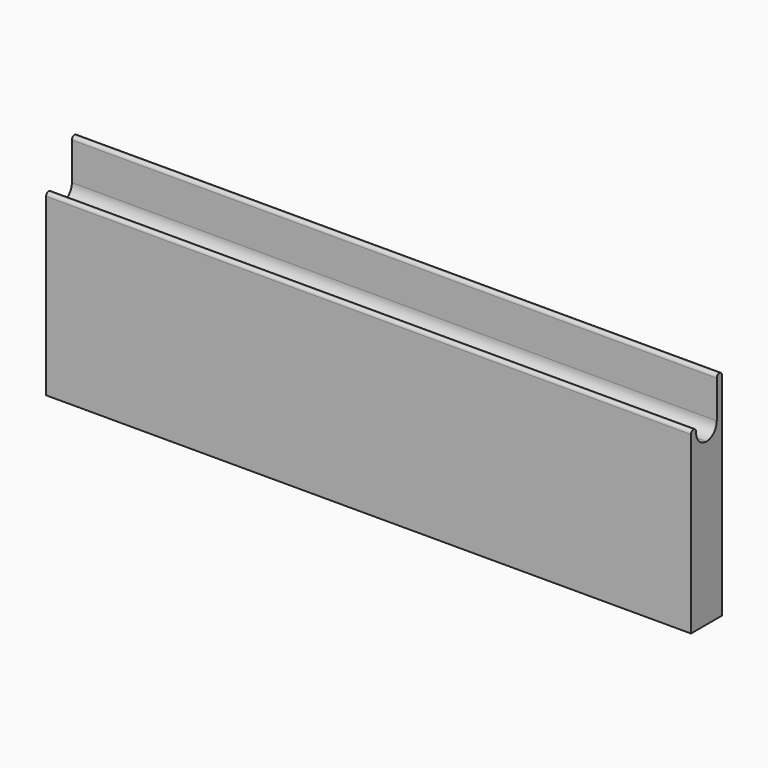
from build123d import *

# Parameters (mm, degrees)
F0_W     = 300
F0_H     = 100
F1_DEPTH = 9
F3_DEPTH = 300.001
F4_R     = 1.49999
F5_R     = 5.99999


# Not quite as in the source:
# - a fillet or chamfer is up to 0.001 mm smaller than in the source, because OpenCascade refuses the exact size


with BuildPart() as f1:
    # F0 (on Front) → F1 (new body, symmetric)
    with BuildSketch(Plane.XZ):
        with Locations((-3.7248600274, -105.7776198197)):
            Rectangle(F0_W, F0_H)
    extrude(amount=F1_DEPTH, both=True)

    # F2 (on face) → F3 (cut, through all)
    with BuildSketch(Plane.YZ.offset(146.2751399726)):
        Polygon((6, -55.7776198197), (-9, -55.7776198197), (-9, -72.7776198197), (-6, -72.7776198197), (-6, -80.7776198197), (6, -80.7776198197), align=None)
    extrude(amount=-F3_DEPTH, mode=Mode.SUBTRACT)

    # F4 (radius 1.5 in the source; OpenCascade refuses exactly that, so slightly less here)
    f4_edges = [f1.edges().sort_by_distance(p)[0] for p in [
        (-3.72486, 6, -55.77762),
        (-3.72486, 9, -55.77762),
        (-3.72486, -9, -72.77762),
        (-3.72486, -6, -72.77762),
    ]]
    fillet(f4_edges, radius=F4_R)

    # F5 (radius 6 in the source; OpenCascade refuses exactly that, so slightly less here)
    f5_edges = [f1.edges().sort_by_distance(p)[0] for p in [
        (-3.72486, 6, -80.77762),
        (-3.72486, -6, -80.77762),
    ]]
    fillet(f5_edges, radius=F5_R)


solid = f1.part
